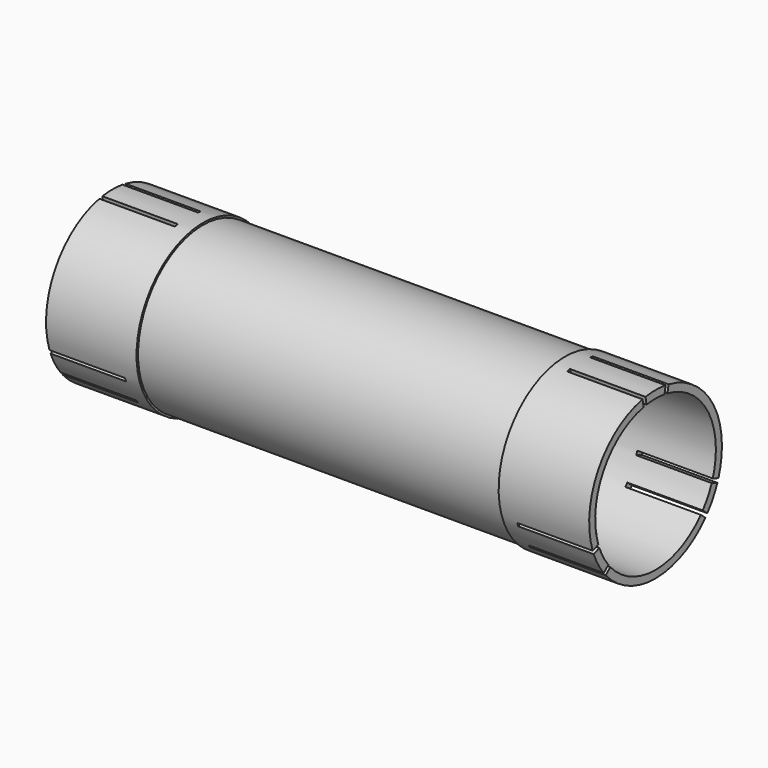
from build123d import *

# Parameters (mm, degrees)
F0_R      = 11
F1_DEPTH  = 12
F2_R      = 10.75
F3_DEPTH  = 48
F4_R      = 11
F4_R_2    = 10.75
F5_DEPTH  = 12
F7_D      = 20
F9_DEPTH  = 10
F11_DEPTH = 10
F14_DEPTH = 5


with BuildPart() as f1:
    # F0 (on Right) → F1 (new body)
    with BuildSketch(Plane.YZ):
        Circle(F0_R)
    extrude(amount=F1_DEPTH)

    # F2 (on face) → F3 (join)
    with BuildSketch(Plane.YZ.offset(12)):
        Circle(F2_R)
    extrude(amount=F3_DEPTH)

    # F4 (on face) → F5 (join)
    with BuildSketch(Plane.YZ.offset(60)):
        Circle(F4_R)
        Circle(F4_R_2, mode=Mode.SUBTRACT)
        Circle(F4_R_2)
    extrude(amount=F5_DEPTH)

    # F7 (through all)
    with Locations(Plane(origin=(0, 0, 0), x_dir=(0, -1, 0), z_dir=(-1, 0, 0))):
        with Locations((0, 0)):
            Hole(F7_D / 2)

    # F8 (on face) → F9 (cut)
    with BuildSketch(Plane(origin=(0, 0, 0), x_dir=(0, -1, 0), z_dir=(-1, 0, 0))):
        with BuildLine():
            Line((1.6634346337, 10.8734992169), (1.5748160855, 10.370918456))
            Line((1.5748160855, 10.370918456), (1.489737103, 9.8884115693))
            ThreePointArc((1.489737103, 9.8884115693), (1.7407460416, 9.8473246732), (1.9906288286, 9.7998671862))
            Line((1.9906288286, 9.7998671862), (2.1643298383, 10.7849745642))
            ThreePointArc((2.1643298383, 10.7849745642), (1.9143939946, 10.8321325524), (1.6634346337, 10.8734992169))
        make_face()
        with BuildLine():
            ThreePointArc((-1.9821409796, 9.8015874805), (-1.7364817767, 9.8480775301), (-1.489737103, 9.8884115693))
            Line((-1.489737103, 9.8884115693), (-1.572378121, 10.3570920718))
            Line((-1.572378121, 10.3570920718), (-1.6634346337, 10.8734992169))
            ThreePointArc((-1.6634346337, 10.8734992169), (-1.9101299543, 10.8328852831), (-2.1558385102, 10.786675128))
            Line((-2.1558385102, 10.786675128), (-2.0647819975, 10.270267983))
            Line((-2.0647819975, 10.270267983), (-1.9821409796, 9.8015874805))
        make_face()
        with BuildLine():
            Line((9.9267039757, -3.3469803284), (9.4794942453, -3.1842092981))
            ThreePointArc((9.4794942453, -3.1842092981), (9.3969262079, -3.4202014333), (9.3084841736, -3.6540556085))
            Line((9.3084841736, -3.6540556085), (9.755693904, -3.8168266388))
            Line((9.755693904, -3.8168266388), (10.2484438667, -3.9961729581))
            ThreePointArc((10.2484438667, -3.9961729581), (10.3366188286, -3.7622215766), (10.4194539383, -3.5263266477))
            Line((10.4194539383, -3.5263266477), (9.9267039757, -3.3469803284))
        make_face()
        with BuildLine():
            ThreePointArc((-9.3084841736, -3.6540556085), (-9.3984063471, -3.416132043), (-9.4822483512, -3.175998458))
            Line((-9.4822483512, -3.175998458), (-10.4222268709, -3.51812266))
            ThreePointArc((-10.4222268709, -3.51812266), (-10.3380989649, -3.758152444), (-10.2484438667, -3.9961729581))
            Line((-10.2484438667, -3.9961729581), (-9.7688868862, -3.8216284916))
            Line((-9.7688868862, -3.8216284916), (-9.3084841736, -3.6540556085))
        make_face()
        with BuildLine():
            Line((8.1940708007, -6.5492899644), (7.8187470706, -6.2343559608))
            ThreePointArc((7.8187470706, -6.2343559608), (7.6576603054, -6.4311926302), (7.4916195226, -6.6238687282))
            Line((7.4916195226, -6.6238687282), (8.2578970327, -7.2668519042))
            ThreePointArc((8.2578970327, -7.2668519042), (8.4237049702, -7.0739801084), (8.585009233, -6.8773262587))
            Line((8.585009233, -6.8773262587), (8.1940708007, -6.5492899644))
        make_face()
        with BuildLine():
            ThreePointArc((-7.4973532657, -6.6173781824), (-7.6604444312, -6.4278760969), (-7.8187470706, -6.2343559608))
            Line((-7.8187470706, -6.2343559608), (-8.1833157831, -6.540265433))
            Line((-8.1833157831, -6.540265433), (-8.585009233, -6.8773262587))
            ThreePointArc((-8.585009233, -6.8773262587), (-8.4264888743, -7.0706637066), (-8.2636154282, -7.2603484803))
            Line((-8.2636154282, -7.2603484803), (-7.8619219782, -6.9232876546))
            Line((-7.8619219782, -6.9232876546), (-7.4973532657, -6.6173781824))
        make_face()
    extrude(amount=-F9_DEPTH, mode=Mode.SUBTRACT)

    # F10 (on face) → F11 (cut)
    with BuildSketch(Plane.YZ.offset(72)):
        with BuildLine():
            ThreePointArc((-1.9821409796, 9.8015874805), (-1.7364817767, 9.8480775301), (-1.489737103, 9.8884115693))
            Line((-1.489737103, 9.8884115693), (-1.6634346337, 10.8734992169))
            ThreePointArc((-1.6634346337, 10.8734992169), (-1.9101299543, 10.8328852831), (-2.1558385102, 10.786675128))
            Line((-2.1558385102, 10.786675128), (-1.9821409796, 9.8015874805))
        make_face()
        with BuildLine():
            Line((1.6634346337, 10.8734992169), (1.489737103, 9.8884115693))
            ThreePointArc((1.489737103, 9.8884115693), (1.7364817767, 9.8480775301), (1.9821409796, 9.8015874805))
            Line((1.9821409796, 9.8015874805), (2.1558385102, 10.786675128))
            ThreePointArc((2.1558385102, 10.786675128), (1.9101299543, 10.8328852831), (1.6634346337, 10.8734992169))
        make_face()
        with BuildLine():
            Line((10.4194539383, -3.5263266477), (9.4794942453, -3.1842092981))
            ThreePointArc((9.4794942453, -3.1842092981), (9.3969262079, -3.4202014333), (9.3084841736, -3.6540556085))
            Line((9.3084841736, -3.6540556085), (10.2484438667, -3.9961729581))
            ThreePointArc((10.2484438667, -3.9961729581), (10.3366188286, -3.7622215766), (10.4194539383, -3.5263266477))
        make_face()
        with BuildLine():
            Line((8.585009233, -6.8773262587), (7.8187470706, -6.2343559608))
            ThreePointArc((7.8187470706, -6.2343559608), (7.6604444312, -6.4278760969), (7.4973532657, -6.6173781824))
            Line((7.4973532657, -6.6173781824), (8.2636154282, -7.2603484803))
            ThreePointArc((8.2636154282, -7.2603484803), (8.4264888743, -7.0706637066), (8.585009233, -6.8773262587))
        make_face()
        with BuildLine():
            ThreePointArc((-9.3084841736, -3.6540556085), (-9.3969262079, -3.4202014333), (-9.4794942453, -3.1842092981))
            Line((-9.4794942453, -3.1842092981), (-10.4194539383, -3.5263266477))
            ThreePointArc((-10.4194539383, -3.5263266477), (-10.3366188286, -3.7622215766), (-10.2484438667, -3.9961729581))
            Line((-10.2484438667, -3.9961729581), (-9.3084841736, -3.6540556085))
        make_face()
        with BuildLine():
            ThreePointArc((-7.4973532657, -6.6173781824), (-7.6604444312, -6.4278760969), (-7.8187470706, -6.2343559608))
            Line((-7.8187470706, -6.2343559608), (-8.585009233, -6.8773262587))
            ThreePointArc((-8.585009233, -6.8773262587), (-8.4264888743, -7.0706637066), (-8.2636154282, -7.2603484803))
            Line((-8.2636154282, -7.2603484803), (-7.4973532657, -6.6173781824))
        make_face()
    extrude(amount=-F11_DEPTH, mode=Mode.SUBTRACT)

    # F13 (on offset) → F14 (cut)
    with BuildSketch(Plane.XY.offset(-11)):
        with BuildLine():
            Line((24, -3.25), (60, -3.25))
            ThreePointArc((60, -3.25), (63.25, 0), (60, 3.25))
            Line((60, 3.25), (24, 3.25))
            ThreePointArc((24, 3.25), (20.75, 0), (24, -3.25))
        make_face()
    extrude(amount=F14_DEPTH, mode=Mode.SUBTRACT)


solid = f1.part
